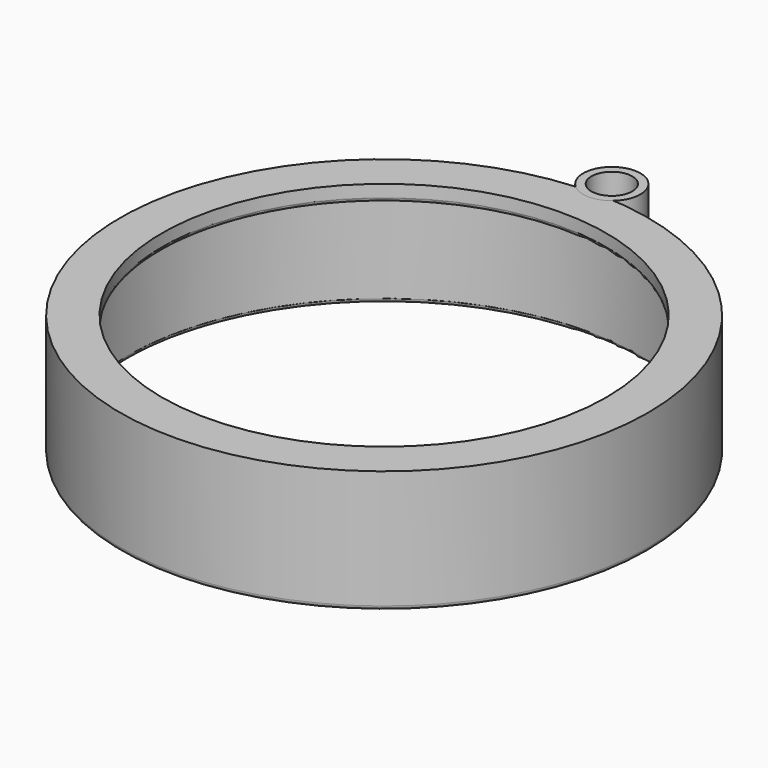
from build123d import *

# Parameters (mm, degrees)
F0_R     = 32.3
F1_DEPTH = 15
F2_R     = 31.3
F3_DEPTH = 13
F4_R     = 27.2
F5_DEPTH = 15
F6_R     = 3.5
F7_DEPTH = 5
F8_R     = 2.5
F9_DEPTH = 5
F12_R    = 0.49999
F12_2_R  = 0.49999


# Not quite as in the source:
# - a fillet or chamfer is up to 0.001 mm smaller than in the source, because OpenCascade refuses the exact size


with BuildPart() as f1:
    # F0 (on Top) → F1 (new body)
    with BuildSketch(Plane.XY):
        Circle(F0_R)
    extrude(amount=F1_DEPTH)

    # F2 (on Top) → F3 (cut)
    with BuildSketch(Plane.XY):
        Circle(F2_R)
    extrude(amount=F3_DEPTH, mode=Mode.SUBTRACT)

    # F4 (on Top) → F5 (cut)
    with BuildSketch(Plane.XY):
        Circle(F4_R)
    extrude(amount=F5_DEPTH, mode=Mode.SUBTRACT)

    # F12 (radius 0.5 in the source; OpenCascade refuses exactly that, so slightly less here)
    f12_edges = [f1.edges().sort_by_distance(p)[0] for p in [
        (-27.2, 0, 13),
        (-31.3, 0, 0),
        (-32.3, 0, 0),
    ]]
    fillet(f12_edges, radius=F12_R)


with BuildPart() as f7:
    # F6 (on Top) → F7 (new body)
    with BuildSketch(Plane.XY):
        Circle(F6_R)
    extrude(amount=F7_DEPTH)

    # F8 (on Top) → F9 (cut)
    with BuildSketch(Plane.XY):
        Circle(F8_R)
    extrude(amount=F9_DEPTH, mode=Mode.SUBTRACT)


with BuildPart() as f7_1:
    # F10: moved
    add(f7.part.moved(Location((0, 34.6, 0))))


with BuildPart() as f7_2:
    # F11: moved
    add(f7_1.part.moved(Location((0, 0.23, 0))))

    # F12#2 (radius 0.5 in the source; OpenCascade refuses exactly that, so slightly less here)
    f12_2_edges = [f7_2.edges().sort_by_distance(p)[0] for p in [
        (-2.5, 34.83, 0),
        (-3.5, 34.83, 0),
    ]]
    fillet(f12_2_edges, radius=F12_2_R)


with BuildPart() as f7_3:
    # F13: moved
    add(f7_2.part.moved(Location((0, 0, 10))))


solid = Compound([f1.part, f7_3.part])
